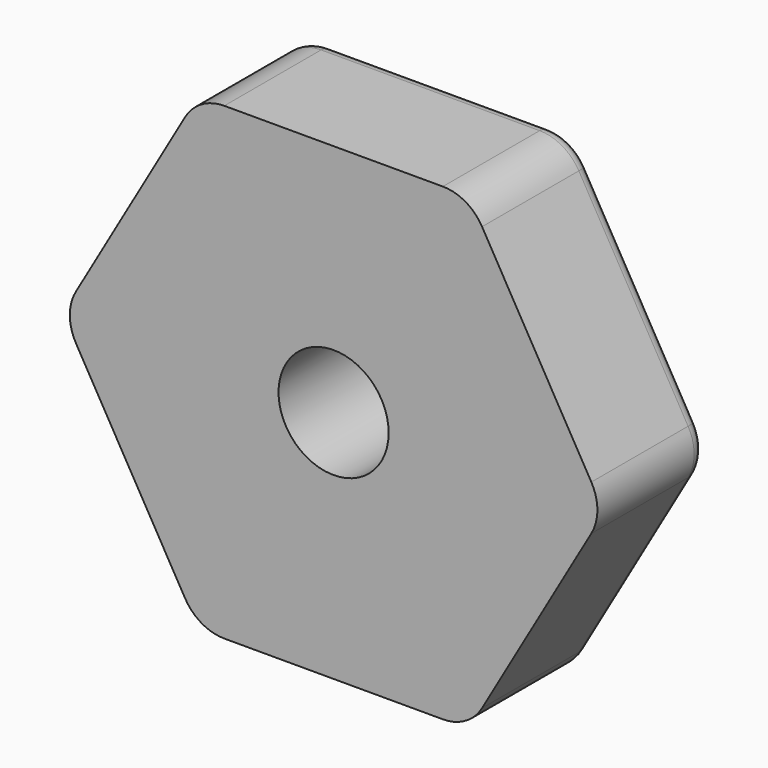
from build123d import *

# Parameters (mm, degrees)
F0_R          = 3.8735
F1_DEPTH      = 9.525
F2_R          = 6.4135
F3_DEPTH      = 6.35
F4_R          = 3.18262
F5_T1_DEPTH   = 5.9170310802
F5_T3_DEPTH   = 5.9170310802
F5_T5_DEPTH   = 5.9170310802
F5_T7_DEPTH   = 5.9170310802
F5_T9_DEPTH   = 5.9170310802
F5_T11_DEPTH  = 5.9170310802
F5_T13_DEPTH  = 5.9170310802
F5_T15_DEPTH  = 5.9170310802
F5_T17_DEPTH  = 5.9170310802
F5_T19_DEPTH  = 5.9170310802
F5_T21_DEPTH  = 5.9170310802
F5_T23_DEPTH  = 5.9170310802
F5_T26_ANGLE  = 76.4394190413
F5_T28_ANGLE  = 16.4394190413
F5_T30_ANGLE  = 16.4394190413
F5_T32_ANGLE  = 76.4394190413
F5_T34_ANGLE  = 76.4394190413
F5_T36_ANGLE  = 16.4394190413
F5_T38_ANGLE  = 16.4394190413
F5_T40_ANGLE  = 76.4394190413
F5_T42_ANGLE  = 76.4394190413
F5_T44_ANGLE  = 16.4394190413
F5_T46_ANGLE  = 16.4394190413
F5_T48_ANGLE  = 76.4394190413
F5_T51_DEPTH  = 15.3750269725
F5_T53_DEPTH  = 15.3750269725
F5_T55_DEPTH  = 15.3750269725
F5_T57_DEPTH  = 15.3750269725
F5_T59_DEPTH  = 15.3750269725
F5_T61_DEPTH  = 5.9170310802
F5_T63_DEPTH  = 5.9170310802
F5_T65_DEPTH  = 5.9170310802
F5_T67_DEPTH  = 5.9170310802
F5_T69_DEPTH  = 5.9170310802
F5_T71_DEPTH  = 5.9170310802
F5_T73_DEPTH  = 5.9170310802
F5_T75_DEPTH  = 5.9170310802
F5_T77_DEPTH  = 5.9170310802
F5_T79_DEPTH  = 5.9170310802
F5_T81_DEPTH  = 5.9170310802
F5_T83_DEPTH  = 5.9170310802
F5_T90_ANGLE  = 76.4394190413
F5_T92_ANGLE  = 60
F5_T94_ANGLE  = 60
F5_T96_ANGLE  = 60
F5_T98_ANGLE  = 60
F5_T100_ANGLE = 60
F5_T102_ANGLE = 60
F5_T104_ANGLE = 16.4394190413
F5_T106_ANGLE = 76.4394190413
F5_T108_ANGLE = 16.4394190413
F5_T110_ANGLE = 76.4394190413
F5_T112_ANGLE = 16.4394190413
F5_T114_ANGLE = 76.4394190413
F5_T116_ANGLE = 16.4394190413
F5_T118_ANGLE = 76.4394190413
F5_T120_ANGLE = 16.4394190413
F5_T122_ANGLE = 76.4394190413
F5_T124_ANGLE = 16.4394190413


# Not quite as in the source:
# - a fillet or chamfer that OpenCascade refuses, or shapes differently, is made with other operations: its cross-section is extruded or revolved along the edge and cut away or added


with BuildPart() as f1:
    # F0 (on Front) → F1 (new body)
    with BuildSketch(Plane.XZ):
        Polygon((19.05, 0), (9.525, 16.4977839421), (-9.525, 16.4977839421), (-19.05, 0), (-9.525, -16.4977839421), (9.525, -16.4977839421), align=None)
        Circle(F0_R, mode=Mode.SUBTRACT)
    extrude(amount=F1_DEPTH)

    # F2 (on face) → F3 (cut)
    with BuildSketch(Plane(origin=(0, 0, 0), x_dir=(-1, 0, 0), z_dir=(0, 1, 0))):
        Polygon((-12.0877954744, 6.978891971), (-17.5835303163, 0), (-12.0877954744, -6.978891971), (-8.7917651581, -15.2277839421), (0, -13.9577839421), (8.7917651581, -15.2277839421), (12.0877954744, -6.978891971), (17.5835303163, 0), (12.0877954744, 6.978891971), (8.7917651581, 15.2277839421), (0, 13.9577839421), (-8.7917651581, 15.2277839421), align=None)
        Circle(F2_R, mode=Mode.SUBTRACT)
    extrude(amount=-F3_DEPTH, mode=Mode.SUBTRACT)

    # F4
    f4_edges = [f1.edges().sort_by_distance(p)[0] for p in [
        (-17.58353, -3.175, 0),
        (-12.087795, -3.175, 6.978892),
        (-8.791765, -3.175, 15.227784),
        (0, -3.175, 13.957784),
        (8.791765, -3.175, 15.227784),
        (12.087795, -3.175, 6.978892),
        (17.58353, -3.175, 0),
        (12.087795, -3.175, -6.978892),
        (8.791765, -3.175, -15.227784),
        (0, -3.175, -13.957784),
        (-8.791765, -3.175, -15.227784),
        (-12.087795, -3.175, -6.978892),
        (-9.525, -4.7625, 16.497784),
        (9.525, -4.7625, 16.497784),
        (19.05, -4.7625, 0),
        (9.525, -4.7625, -16.497784),
        (-19.05, -4.7625, 0),
        (-9.525, -4.7625, -16.497784),
    ]]
    fillet(f4_edges, radius=F4_R)

    # F5: fillet of radius 1.016 on 29 edges, made by hand

    # F5_s2 → F5_t1 (join)
    with BuildSketch(Plane(origin=(-8.286299479, 0, 1.1969837853), x_dir=(0, 1, 0), z_dir=(0.9897271086, 0, -0.1429694044))):
        with BuildLine():
            ThreePointArc((-5.334, 13.8143971429), (-6.0524204897, 13.5168176326), (-6.35, 12.7983971429))
            Line((-6.35, 12.7983971429), (-6.35, 13.8143971429))
            Line((-6.35, 13.8143971429), (-5.334, 13.8143971429))
        make_face()
    extrude(amount=F5_T1_DEPTH)

    # F5_s4 → F5_t3 (join)
    with BuildSketch(Plane(origin=(0.9110263511, 0, 2.2800026795), x_dir=(0, 1, 0), z_dir=(0.3710484181, 0, 0.928613521))):
        with BuildLine():
            ThreePointArc((-5.334, 13.8143971429), (-6.0524204897, 13.5168176326), (-6.35, 12.7983971429))
            Line((-6.35, 12.7983971429), (-6.35, 13.8143971429))
            Line((-6.35, 13.8143971429), (-5.334, 13.8143971429))
        make_face()
    extrude(amount=F5_T3_DEPTH)

    # F5_s6 → F5_t5 (join)
    with BuildSketch(Plane(origin=(2.4300534167, 0, 0.3510293762), x_dir=(0, 1, 0), z_dir=(0.9897271086, 0, 0.1429694044))):
        with BuildLine():
            ThreePointArc((-5.334, 13.8143971429), (-6.0524204897, 13.5168176326), (-6.35, 12.7983971429))
            Line((-6.35, 12.7983971429), (-6.35, 13.8143971429))
            Line((-6.35, 13.8143971429), (-5.334, 13.8143971429))
        make_face()
    extrude(amount=F5_T5_DEPTH)

    # F5_s8 → F5_t7 (join)
    with BuildSketch(Plane(origin=(-5.1797681055, 0, -6.5776539596), x_dir=(0, 1, 0), z_dir=(0.6186786904, 0, 0.7856441167))):
        with BuildLine():
            ThreePointArc((-5.334, 13.8143971429), (-6.0524204897, 13.5168176326), (-6.35, 12.7983971429))
            Line((-6.35, 12.7983971429), (-6.35, 13.8143971429))
            Line((-6.35, 13.8143971429), (-5.334, 13.8143971429))
        make_face()
    extrude(amount=F5_T7_DEPTH)

    # F5_s10 → F5_t9 (join)
    with BuildSketch(Plane(origin=(-3.1065313735, 0, 7.7746377448), x_dir=(0, 1, 0), z_dir=(0.3710484181, 0, -0.928613521))):
        with BuildLine():
            ThreePointArc((-5.334, 13.8143971429), (-6.0524204897, 13.5168176326), (-6.35, 12.7983971429))
            Line((-6.35, 12.7983971429), (-6.35, 13.8143971429))
            Line((-6.35, 13.8143971429), (-5.334, 13.8143971429))
        make_face()
    extrude(amount=F5_T9_DEPTH)

    # F5_s12 → F5_t11 (join)
    with BuildSketch(Plane(origin=(-1.5190270656, 0, 1.9289733033), x_dir=(0, 1, 0), z_dir=(-0.6186786904, 0, 0.7856441167))):
        with BuildLine():
            ThreePointArc((-5.334, 13.8143971429), (-6.0524204897, 13.5168176326), (-6.35, 12.7983971429))
            Line((-6.35, 12.7983971429), (-6.35, 13.8143971429))
            Line((-6.35, 13.8143971429), (-5.334, 13.8143971429))
        make_face()
    extrude(amount=F5_T11_DEPTH)

    # F5_s14 → F5_t13 (join)
    with BuildSketch(Plane(origin=(1.5190270656, 0, -1.9289733033), x_dir=(0, 1, 0), z_dir=(0.6186786904, 0, -0.7856441167))):
        with BuildLine():
            ThreePointArc((-5.334, 13.8143971429), (-6.0524204897, 13.5168176326), (-6.35, 12.7983971429))
            Line((-6.35, 12.7983971429), (-6.35, 13.8143971429))
            Line((-6.35, 13.8143971429), (-5.334, 13.8143971429))
        make_face()
    extrude(amount=F5_T13_DEPTH)

    # F5_s16 → F5_t15 (join)
    with BuildSketch(Plane(origin=(3.1065313735, 0, -7.7746377448), x_dir=(0, 1, 0), z_dir=(-0.3710484181, 0, 0.928613521))):
        with BuildLine():
            ThreePointArc((-5.334, 13.8143971429), (-6.0524204897, 13.5168176326), (-6.35, 12.7983971429))
            Line((-6.35, 12.7983971429), (-6.35, 13.8143971429))
            Line((-6.35, 13.8143971429), (-5.334, 13.8143971429))
        make_face()
    extrude(amount=F5_T15_DEPTH)

    # F5_s18 → F5_t17 (join)
    with BuildSketch(Plane(origin=(5.1797681055, 0, 6.5776539596), x_dir=(0, 1, 0), z_dir=(-0.6186786904, 0, -0.7856441167))):
        with BuildLine():
            ThreePointArc((-5.334, 13.8143971429), (-6.0524204897, 13.5168176326), (-6.35, 12.7983971429))
            Line((-6.35, 12.7983971429), (-6.35, 13.8143971429))
            Line((-6.35, 13.8143971429), (-5.334, 13.8143971429))
        make_face()
    extrude(amount=F5_T17_DEPTH)

    # F5_s20 → F5_t19 (join)
    with BuildSketch(Plane(origin=(-2.4300534167, 0, -0.3510293762), x_dir=(0, 1, 0), z_dir=(-0.9897271086, 0, -0.1429694044))):
        with BuildLine():
            ThreePointArc((-5.334, 13.8143971429), (-6.0524204897, 13.5168176326), (-6.35, 12.7983971429))
            Line((-6.35, 12.7983971429), (-6.35, 13.8143971429))
            Line((-6.35, 13.8143971429), (-5.334, 13.8143971429))
        make_face()
    extrude(amount=F5_T19_DEPTH)

    # F5_s22 → F5_t21 (join)
    with BuildSketch(Plane(origin=(-0.9110263511, 0, -2.2800026795), x_dir=(0, 1, 0), z_dir=(-0.3710484181, 0, -0.928613521))):
        with BuildLine():
            ThreePointArc((-5.334, 13.8143971429), (-6.0524204897, 13.5168176326), (-6.35, 12.7983971429))
            Line((-6.35, 12.7983971429), (-6.35, 13.8143971429))
            Line((-6.35, 13.8143971429), (-5.334, 13.8143971429))
        make_face()
    extrude(amount=F5_T21_DEPTH)

    # F5_s24 → F5_t23 (join)
    with BuildSketch(Plane(origin=(8.286299479, 0, -1.1969837853), x_dir=(0, 1, 0), z_dir=(-0.9897271086, 0, 0.1429694044))):
        with BuildLine():
            ThreePointArc((-5.334, 13.8143971429), (-6.0524204897, 13.5168176326), (-6.35, 12.7983971429))
            Line((-6.35, 12.7983971429), (-6.35, 13.8143971429))
            Line((-6.35, 13.8143971429), (-5.334, 13.8143971429))
        make_face()
    extrude(amount=F5_T23_DEPTH)

    # F5_s25 → F5_t26 (revolve)
    with BuildSketch(Plane(origin=(3.1065313735, 0, 7.7746377448), x_dir=(0, 1, 0), z_dir=(-0.3710484181, 0, -0.928613521))):
        with BuildLine():
            ThreePointArc((-5.334, -13.8143971429), (-6.0524204897, -13.5168176326), (-6.35, -12.7983971429))
            Line((-6.35, -12.7983971429), (-6.35, -13.8143971429))
            Line((-6.35, -13.8143971429), (-5.334, -13.8143971429))
        make_face()
    revolve(axis=Axis((-6.7662806337, -6.35, 11.7195418358), (0, 1, 0)), revolution_arc=F5_T26_ANGLE)

    # F5_s27 → F5_t28 (revolve)
    with BuildSketch(Plane(origin=(2.4300534167, 0, 0.3510293762), x_dir=(0, 1, 0), z_dir=(0.9897271086, 0, 0.1429694044))):
        with BuildLine():
            ThreePointArc((-5.334, 13.8143971429), (-6.0524204897, 13.5168176326), (-6.35, 12.7983971429))
            Line((-6.35, 12.7983971429), (-6.35, 13.8143971429))
            Line((-6.35, 13.8143971429), (-5.334, 13.8143971429))
        make_face()
    revolve(axis=Axis((0, -6.35, 17.1734380072), (0, 1, 0)), revolution_arc=F5_T28_ANGLE)

    # F5_s29 → F5_t30 (revolve)
    with BuildSketch(Plane(origin=(0.9110263511, 0, 2.2800026795), x_dir=(0, 1, 0), z_dir=(0.3710484181, 0, 0.928613521))):
        with BuildLine():
            ThreePointArc((-5.334, 13.8143971429), (-6.0524204897, 13.5168176326), (-6.35, 12.7983971429))
            Line((-6.35, 12.7983971429), (-6.35, 13.8143971429))
            Line((-6.35, 13.8143971429), (-5.334, 13.8143971429))
        make_face()
    revolve(axis=Axis((-14.8726335846, -6.35, 8.5867190036), (0, 1, 0)), revolution_arc=F5_T30_ANGLE)

    # F5_s31 → F5_t32 (revolve)
    with BuildSketch(Plane(origin=(-3.1065313735, 0, 7.7746377448), x_dir=(0, 1, 0), z_dir=(0.3710484181, 0, -0.928613521))):
        with BuildLine():
            ThreePointArc((-5.334, 13.8143971429), (-6.0524204897, 13.5168176326), (-6.35, 12.7983971429))
            Line((-6.35, 12.7983971429), (-6.35, 13.8143971429))
            Line((-6.35, 13.8143971429), (-5.334, 13.8143971429))
        make_face()
    revolve(axis=Axis((6.7662806337, -6.35, 11.7195418358), (0, -1, 0)), revolution_arc=F5_T32_ANGLE)

    # F5_s33 → F5_t34 (revolve)
    with BuildSketch(Plane(origin=(-5.1797681055, 0, -6.5776539596), x_dir=(0, 1, 0), z_dir=(0.6186786904, 0, 0.7856441167))):
        with BuildLine():
            ThreePointArc((-5.334, 13.8143971429), (-6.0524204897, 13.5168176326), (-6.35, 12.7983971429))
            Line((-6.35, 12.7983971429), (-6.35, 13.8143971429))
            Line((-6.35, 13.8143971429), (-5.334, 13.8143971429))
        make_face()
    revolve(axis=Axis((-13.5325612674, -6.35, 0), (0, -1, 0)), revolution_arc=F5_T34_ANGLE)

    # F5_s35 → F5_t36 (revolve)
    with BuildSketch(Plane(origin=(1.5190270656, 0, -1.9289733033), x_dir=(0, 1, 0), z_dir=(0.6186786904, 0, -0.7856441167))):
        with BuildLine():
            ThreePointArc((-5.334, 13.8143971429), (-6.0524204897, 13.5168176326), (-6.35, 12.7983971429))
            Line((-6.35, 12.7983971429), (-6.35, 13.8143971429))
            Line((-6.35, 13.8143971429), (-5.334, 13.8143971429))
        make_face()
    revolve(axis=Axis((14.8726335846, -6.35, 8.5867190036), (0, 1, 0)), revolution_arc=F5_T36_ANGLE)

    # F5_s37 → F5_t38 (revolve)
    with BuildSketch(Plane(origin=(-1.5190270656, 0, 1.9289733033), x_dir=(0, 1, 0), z_dir=(-0.6186786904, 0, 0.7856441167))):
        with BuildLine():
            ThreePointArc((-5.334, 13.8143971429), (-6.0524204897, 13.5168176326), (-6.35, 12.7983971429))
            Line((-6.35, 12.7983971429), (-6.35, 13.8143971429))
            Line((-6.35, 13.8143971429), (-5.334, 13.8143971429))
        make_face()
    revolve(axis=Axis((-14.8726335846, -6.35, -8.5867190036), (0, 1, 0)), revolution_arc=F5_T38_ANGLE)

    # F5_s39 → F5_t40 (revolve)
    with BuildSketch(Plane(origin=(5.1797681055, 0, 6.5776539596), x_dir=(0, 1, 0), z_dir=(-0.6186786904, 0, -0.7856441167))):
        with BuildLine():
            ThreePointArc((-5.334, 13.8143971429), (-6.0524204897, 13.5168176326), (-6.35, 12.7983971429))
            Line((-6.35, 12.7983971429), (-6.35, 13.8143971429))
            Line((-6.35, 13.8143971429), (-5.334, 13.8143971429))
        make_face()
    revolve(axis=Axis((13.5325612674, -6.35, 0), (0, -1, 0)), revolution_arc=F5_T40_ANGLE)

    # F5_s41 → F5_t42 (revolve)
    with BuildSketch(Plane(origin=(3.1065313735, 0, -7.7746377448), x_dir=(0, 1, 0), z_dir=(-0.3710484181, 0, 0.928613521))):
        with BuildLine():
            ThreePointArc((-5.334, 13.8143971429), (-6.0524204897, 13.5168176326), (-6.35, 12.7983971429))
            Line((-6.35, 12.7983971429), (-6.35, 13.8143971429))
            Line((-6.35, 13.8143971429), (-5.334, 13.8143971429))
        make_face()
    revolve(axis=Axis((-6.7662806337, -6.35, -11.7195418358), (0, -1, 0)), revolution_arc=F5_T42_ANGLE)

    # F5_s43 → F5_t44 (revolve)
    with BuildSketch(Plane(origin=(-0.9110263511, 0, -2.2800026795), x_dir=(0, 1, 0), z_dir=(-0.3710484181, 0, -0.928613521))):
        with BuildLine():
            ThreePointArc((-5.334, 13.8143971429), (-6.0524204897, 13.5168176326), (-6.35, 12.7983971429))
            Line((-6.35, 12.7983971429), (-6.35, 13.8143971429))
            Line((-6.35, 13.8143971429), (-5.334, 13.8143971429))
        make_face()
    revolve(axis=Axis((14.8726335846, -6.35, -8.5867190036), (0, 1, 0)), revolution_arc=F5_T44_ANGLE)

    # F5_s45 → F5_t46 (revolve)
    with BuildSketch(Plane(origin=(-2.4300534167, 0, -0.3510293762), x_dir=(0, 1, 0), z_dir=(-0.9897271086, 0, -0.1429694044))):
        with BuildLine():
            ThreePointArc((-5.334, 13.8143971429), (-6.0524204897, 13.5168176326), (-6.35, 12.7983971429))
            Line((-6.35, 12.7983971429), (-6.35, 13.8143971429))
            Line((-6.35, 13.8143971429), (-5.334, 13.8143971429))
        make_face()
    revolve(axis=Axis((0, -6.35, -17.1734380072), (0, 1, 0)), revolution_arc=F5_T46_ANGLE)

    # F5_s47 → F5_t48 (revolve)
    with BuildSketch(Plane(origin=(8.286299479, 0, -1.1969837853), x_dir=(0, 1, 0), z_dir=(-0.9897271086, 0, 0.1429694044))):
        with BuildLine():
            ThreePointArc((-5.334, 13.8143971429), (-6.0524204897, 13.5168176326), (-6.35, 12.7983971429))
            Line((-6.35, 12.7983971429), (-6.35, 13.8143971429))
            Line((-6.35, 13.8143971429), (-5.334, 13.8143971429))
        make_face()
    revolve(axis=Axis((6.7662806337, -6.35, -11.7195418358), (0, -1, 0)), revolution_arc=F5_T48_ANGLE)

    # F5_s49 → F5_t50 (revolve)
    with BuildSketch(Plane.XY):
        with BuildLine():
            ThreePointArc((-7.4295, -6.35), (-6.7110795103, -6.0524204897), (-6.4135, -5.334))
            Line((-6.4135, -5.334), (-6.4135, -6.35))
            Line((-6.4135, -6.35), (-7.4295, -6.35))
        make_face()
    revolve(axis=Axis((0, -6.35, 0), (0, 1, 0)))

    # F5_s52 → F5_t51 (cut)
    with BuildSketch(Plane(origin=(-3.8437567431, 0, -6.657581971), x_dir=(0, 1, 0), z_dir=(0.5, 0, 0.8660254038))):
        with BuildLine():
            ThreePointArc((-1.016, -16.4977839421), (-0.2975795103, -16.2002044318), (0, -15.4817839421))
            Line((0, -15.4817839421), (0, -16.4977839421))
            Line((0, -16.4977839421), (-1.016, -16.4977839421))
        make_face()
    extrude(amount=F5_T51_DEPTH, mode=Mode.SUBTRACT)

    # F5_s54 → F5_t53 (cut)
    with BuildSketch(Plane(origin=(3.8437567431, 0, -6.657581971), x_dir=(0, 1, 0), z_dir=(-0.5, 0, 0.8660254038))):
        with BuildLine():
            ThreePointArc((0, -15.4817839421), (-0.2975795103, -16.2002044318), (-1.016, -16.4977839421))
            Line((-1.016, -16.4977839421), (0, -16.4977839421))
            Line((0, -16.4977839421), (0, -15.4817839421))
        make_face()
    extrude(amount=F5_T53_DEPTH, mode=Mode.SUBTRACT)

    # F5_s56 → F5_t55 (cut)
    with BuildSketch(Plane.YZ.offset(-7.6875134863)):
        with BuildLine():
            ThreePointArc((0, 15.4817839421), (-0.2975795103, 16.2002044318), (-1.016, 16.4977839421))
            Line((-1.016, 16.4977839421), (0, 16.4977839421))
            Line((0, 16.4977839421), (0, 15.4817839421))
        make_face()
        with BuildLine():
            ThreePointArc((0, -15.4817839421), (-0.2975795103, -16.2002044318), (-1.016, -16.4977839421))
            Line((-1.016, -16.4977839421), (0, -16.4977839421))
            Line((0, -16.4977839421), (0, -15.4817839421))
        make_face()
    extrude(amount=F5_T55_DEPTH, mode=Mode.SUBTRACT)

    # F5_s58 → F5_t57 (cut)
    with BuildSketch(Plane(origin=(3.8437567431, 0, 6.657581971), x_dir=(0, 1, 0), z_dir=(-0.5, 0, -0.8660254038))):
        with BuildLine():
            ThreePointArc((0, -15.4817839421), (-0.2975795103, -16.2002044318), (-1.016, -16.4977839421))
            Line((-1.016, -16.4977839421), (0, -16.4977839421))
            Line((0, -16.4977839421), (0, -15.4817839421))
        make_face()
    extrude(amount=F5_T57_DEPTH, mode=Mode.SUBTRACT)

    # F5_s60 → F5_t59 (cut)
    with BuildSketch(Plane(origin=(-3.8437567431, 0, 6.657581971), x_dir=(0, 1, 0), z_dir=(0.5, 0, -0.8660254038))):
        with BuildLine():
            ThreePointArc((0, -15.4817839421), (-0.2975795103, -16.2002044318), (-1.016, -16.4977839421))
            Line((-1.016, -16.4977839421), (0, -16.4977839421))
            Line((0, -16.4977839421), (0, -15.4817839421))
        make_face()
    extrude(amount=F5_T59_DEPTH, mode=Mode.SUBTRACT)

    # F5_s62 → F5_t61 (cut)
    with BuildSketch(Plane(origin=(5.1797681055, 0, 6.5776539596), x_dir=(0, 1, 0), z_dir=(-0.6186786904, 0, -0.7856441167))):
        with BuildLine():
            ThreePointArc((0, 14.8303971429), (-0.2975795103, 14.1119766532), (-1.016, 13.8143971429))
            Line((-1.016, 13.8143971429), (0, 13.8143971429))
            Line((0, 13.8143971429), (0, 14.8303971429))
        make_face()
    extrude(amount=F5_T61_DEPTH, mode=Mode.SUBTRACT)

    # F5_s64 → F5_t63 (cut)
    with BuildSketch(Plane(origin=(1.5190270656, 0, -1.9289733033), x_dir=(0, 1, 0), z_dir=(0.6186786904, 0, -0.7856441167))):
        with BuildLine():
            ThreePointArc((0, 14.8303971429), (-0.2975795103, 14.1119766532), (-1.016, 13.8143971429))
            Line((-1.016, 13.8143971429), (0, 13.8143971429))
            Line((0, 13.8143971429), (0, 14.8303971429))
        make_face()
    extrude(amount=F5_T63_DEPTH, mode=Mode.SUBTRACT)

    # F5_s66 → F5_t65 (cut)
    with BuildSketch(Plane(origin=(-3.1065313735, 0, 7.7746377448), x_dir=(0, 1, 0), z_dir=(0.3710484181, 0, -0.928613521))):
        with BuildLine():
            ThreePointArc((0, 14.8303971429), (-0.2975795103, 14.1119766532), (-1.016, 13.8143971429))
            Line((-1.016, 13.8143971429), (0, 13.8143971429))
            Line((0, 13.8143971429), (0, 14.8303971429))
        make_face()
    extrude(amount=F5_T65_DEPTH, mode=Mode.SUBTRACT)

    # F5_s68 → F5_t67 (cut)
    with BuildSketch(Plane(origin=(2.4300534167, 0, 0.3510293762), x_dir=(0, 1, 0), z_dir=(0.9897271086, 0, 0.1429694044))):
        with BuildLine():
            ThreePointArc((0, 14.8303971429), (-0.2975795103, 14.1119766532), (-1.016, 13.8143971429))
            Line((-1.016, 13.8143971429), (0, 13.8143971429))
            Line((0, 13.8143971429), (0, 14.8303971429))
        make_face()
    extrude(amount=F5_T67_DEPTH, mode=Mode.SUBTRACT)

    # F5_s70 → F5_t69 (cut)
    with BuildSketch(Plane(origin=(-8.286299479, 0, 1.1969837853), x_dir=(0, 1, 0), z_dir=(0.9897271086, 0, -0.1429694044))):
        with BuildLine():
            ThreePointArc((0, 14.8303971429), (-0.2975795103, 14.1119766532), (-1.016, 13.8143971429))
            Line((-1.016, 13.8143971429), (0, 13.8143971429))
            Line((0, 13.8143971429), (0, 14.8303971429))
        make_face()
    extrude(amount=F5_T69_DEPTH, mode=Mode.SUBTRACT)

    # F5_s72 → F5_t71 (cut)
    with BuildSketch(Plane(origin=(0.9110263511, 0, 2.2800026795), x_dir=(0, 1, 0), z_dir=(0.3710484181, 0, 0.928613521))):
        with BuildLine():
            ThreePointArc((0, 14.8303971429), (-0.2975795103, 14.1119766532), (-1.016, 13.8143971429))
            Line((-1.016, 13.8143971429), (0, 13.8143971429))
            Line((0, 13.8143971429), (0, 14.8303971429))
        make_face()
    extrude(amount=F5_T71_DEPTH, mode=Mode.SUBTRACT)

    # F5_s74 → F5_t73 (cut)
    with BuildSketch(Plane(origin=(-5.1797681055, 0, -6.5776539596), x_dir=(0, 1, 0), z_dir=(0.6186786904, 0, 0.7856441167))):
        with BuildLine():
            ThreePointArc((0, 14.8303971429), (-0.2975795103, 14.1119766532), (-1.016, 13.8143971429))
            Line((-1.016, 13.8143971429), (0, 13.8143971429))
            Line((0, 13.8143971429), (0, 14.8303971429))
        make_face()
    extrude(amount=F5_T73_DEPTH, mode=Mode.SUBTRACT)

    # F5_s76 → F5_t75 (cut)
    with BuildSketch(Plane(origin=(-1.5190270656, 0, 1.9289733033), x_dir=(0, 1, 0), z_dir=(-0.6186786904, 0, 0.7856441167))):
        with BuildLine():
            ThreePointArc((0, 14.8303971429), (-0.2975795103, 14.1119766532), (-1.016, 13.8143971429))
            Line((-1.016, 13.8143971429), (0, 13.8143971429))
            Line((0, 13.8143971429), (0, 14.8303971429))
        make_face()
    extrude(amount=F5_T75_DEPTH, mode=Mode.SUBTRACT)

    # F5_s78 → F5_t77 (cut)
    with BuildSketch(Plane(origin=(3.1065313735, 0, -7.7746377448), x_dir=(0, 1, 0), z_dir=(-0.3710484181, 0, 0.928613521))):
        with BuildLine():
            ThreePointArc((0, 14.8303971429), (-0.2975795103, 14.1119766532), (-1.016, 13.8143971429))
            Line((-1.016, 13.8143971429), (0, 13.8143971429))
            Line((0, 13.8143971429), (0, 14.8303971429))
        make_face()
    extrude(amount=F5_T77_DEPTH, mode=Mode.SUBTRACT)

    # F5_s80 → F5_t79 (cut)
    with BuildSketch(Plane(origin=(-2.4300534167, 0, -0.3510293762), x_dir=(0, 1, 0), z_dir=(-0.9897271086, 0, -0.1429694044))):
        with BuildLine():
            ThreePointArc((0, 14.8303971429), (-0.2975795103, 14.1119766532), (-1.016, 13.8143971429))
            Line((-1.016, 13.8143971429), (0, 13.8143971429))
            Line((0, 13.8143971429), (0, 14.8303971429))
        make_face()
    extrude(amount=F5_T79_DEPTH, mode=Mode.SUBTRACT)

    # F5_s82 → F5_t81 (cut)
    with BuildSketch(Plane(origin=(8.286299479, 0, -1.1969837853), x_dir=(0, 1, 0), z_dir=(-0.9897271086, 0, 0.1429694044))):
        with BuildLine():
            ThreePointArc((0, 14.8303971429), (-0.2975795103, 14.1119766532), (-1.016, 13.8143971429))
            Line((-1.016, 13.8143971429), (0, 13.8143971429))
            Line((0, 13.8143971429), (0, 14.8303971429))
        make_face()
    extrude(amount=F5_T81_DEPTH, mode=Mode.SUBTRACT)

    # F5_s84 → F5_t83 (cut)
    with BuildSketch(Plane(origin=(-0.9110263511, 0, -2.2800026795), x_dir=(0, 1, 0), z_dir=(-0.3710484181, 0, -0.928613521))):
        with BuildLine():
            ThreePointArc((0, 14.8303971429), (-0.2975795103, 14.1119766532), (-1.016, 13.8143971429))
            Line((-1.016, 13.8143971429), (0, 13.8143971429))
            Line((0, 13.8143971429), (0, 14.8303971429))
        make_face()
    extrude(amount=F5_T83_DEPTH, mode=Mode.SUBTRACT)

    # F5_s85 → F5_t86 (revolve, cut)
    with BuildSketch(Plane.XY):
        with BuildLine():
            ThreePointArc((-5.3975, 0), (-6.1159204897, -0.2975795103), (-6.4135, -1.016))
            Line((-6.4135, -1.016), (-6.4135, 0))
            Line((-6.4135, 0), (-5.3975, 0))
        make_face()
    revolve(axis=Axis((0, 0, 0), (0, 1, 0)), mode=Mode.SUBTRACT)

    # F5_s87 → F5_t88 (revolve, cut)
    with BuildSketch(Plane.XY):
        with BuildLine():
            ThreePointArc((3.8735, -1.016), (4.1710795103, -0.2975795103), (4.8895, 0))
            Line((4.8895, 0), (3.8735, 0))
            Line((3.8735, 0), (3.8735, -1.016))
        make_face()
    revolve(axis=Axis((0, 0, 0), (0, -1, 0)), mode=Mode.SUBTRACT)

    # F5_s89 → F5_t90 (revolve, cut)
    with BuildSketch(Plane(origin=(5.1797681055, 0, 6.5776539596), x_dir=(0, 1, 0), z_dir=(-0.6186786904, 0, -0.7856441167))):
        with BuildLine():
            ThreePointArc((0, 14.8303971429), (-0.2975795103, 14.1119766532), (-1.016, 13.8143971429))
            Line((-1.016, 13.8143971429), (0, 13.8143971429))
            Line((0, 13.8143971429), (0, 14.8303971429))
        make_face()
    revolve(axis=Axis((13.5325612674, 0, 0), (0, -1, 0)), revolution_arc=F5_T90_ANGLE, mode=Mode.SUBTRACT)

    # F5_s91 → F5_t92 (revolve, cut)
    with BuildSketch(Plane(origin=(3.8437567431, 0, 6.657581971), x_dir=(0, 1, 0), z_dir=(-0.5, 0, -0.8660254038))):
        with BuildLine():
            ThreePointArc((0, 15.4817839421), (-0.2975795103, 16.2002044318), (-1.016, 16.4977839421))
            Line((-1.016, 16.4977839421), (0, 16.4977839421))
            Line((0, 16.4977839421), (0, 15.4817839421))
        make_face()
    revolve(axis=Axis((15.3750269725, 0, 0), (0, -1, 0)), revolution_arc=F5_T92_ANGLE, mode=Mode.SUBTRACT)

    # F5_s93 → F5_t94 (revolve, cut)
    with BuildSketch(Plane(origin=(-3.8437567431, 0, 6.657581971), x_dir=(0, 1, 0), z_dir=(0.5, 0, -0.8660254038))):
        with BuildLine():
            ThreePointArc((0, 15.4817839421), (-0.2975795103, 16.2002044318), (-1.016, 16.4977839421))
            Line((-1.016, 16.4977839421), (0, 16.4977839421))
            Line((0, 16.4977839421), (0, 15.4817839421))
        make_face()
    revolve(axis=Axis((7.6875134863, 0, 13.3151639421), (0, -1, 0)), revolution_arc=F5_T94_ANGLE, mode=Mode.SUBTRACT)

    # F5_s95 → F5_t96 (revolve, cut)
    with BuildSketch(Plane.YZ.offset(-7.6875134863)):
        with BuildLine():
            ThreePointArc((0, 15.4817839421), (-0.2975795103, 16.2002044318), (-1.016, 16.4977839421))
            Line((-1.016, 16.4977839421), (0, 16.4977839421))
            Line((0, 16.4977839421), (0, 15.4817839421))
        make_face()
    revolve(axis=Axis((-7.6875134863, 0, 13.3151639421), (0, -1, 0)), revolution_arc=F5_T96_ANGLE, mode=Mode.SUBTRACT)

    # F5_s97 → F5_t98 (revolve, cut)
    with BuildSketch(Plane(origin=(-3.8437567431, 0, 6.657581971), x_dir=(0, 1, 0), z_dir=(0.5, 0, -0.8660254038))):
        with BuildLine():
            ThreePointArc((0, -15.4817839421), (-0.2975795103, -16.2002044318), (-1.016, -16.4977839421))
            Line((-1.016, -16.4977839421), (0, -16.4977839421))
            Line((0, -16.4977839421), (0, -15.4817839421))
        make_face()
    revolve(axis=Axis((-15.3750269725, 0, 0), (0, 1, 0)), revolution_arc=F5_T98_ANGLE, mode=Mode.SUBTRACT)

    # F5_s99 → F5_t100 (revolve, cut)
    with BuildSketch(Plane.YZ.offset(-7.6875134863)):
        with BuildLine():
            ThreePointArc((0, -15.4817839421), (-0.2975795103, -16.2002044318), (-1.016, -16.4977839421))
            Line((-1.016, -16.4977839421), (0, -16.4977839421))
            Line((0, -16.4977839421), (0, -15.4817839421))
        make_face()
    revolve(axis=Axis((-7.6875134863, 0, -13.3151639421), (0, 1, 0)), revolution_arc=F5_T100_ANGLE, mode=Mode.SUBTRACT)

    # F5_s101 → F5_t102 (revolve, cut)
    with BuildSketch(Plane(origin=(-3.8437567431, 0, -6.657581971), x_dir=(0, 1, 0), z_dir=(0.5, 0, 0.8660254038))):
        with BuildLine():
            ThreePointArc((0, -15.4817839421), (-0.2975795103, -16.2002044318), (-1.016, -16.4977839421))
            Line((-1.016, -16.4977839421), (0, -16.4977839421))
            Line((0, -16.4977839421), (0, -15.4817839421))
        make_face()
    revolve(axis=Axis((7.6875134863, 0, -13.3151639421), (0, 1, 0)), revolution_arc=F5_T102_ANGLE, mode=Mode.SUBTRACT)

    # F5_s103 → F5_t104 (revolve, cut)
    with BuildSketch(Plane(origin=(1.5190270656, 0, -1.9289733033), x_dir=(0, 1, 0), z_dir=(0.6186786904, 0, -0.7856441167))):
        with BuildLine():
            ThreePointArc((0, 14.8303971429), (-0.2975795103, 14.1119766532), (-1.016, 13.8143971429))
            Line((-1.016, 13.8143971429), (0, 13.8143971429))
            Line((0, 13.8143971429), (0, 14.8303971429))
        make_face()
    revolve(axis=Axis((14.8726335846, 0, 8.5867190036), (0, 1, 0)), revolution_arc=F5_T104_ANGLE, mode=Mode.SUBTRACT)

    # F5_s105 → F5_t106 (revolve, cut)
    with BuildSketch(Plane(origin=(-3.1065313735, 0, 7.7746377448), x_dir=(0, 1, 0), z_dir=(0.3710484181, 0, -0.928613521))):
        with BuildLine():
            ThreePointArc((0, 14.8303971429), (-0.2975795103, 14.1119766532), (-1.016, 13.8143971429))
            Line((-1.016, 13.8143971429), (0, 13.8143971429))
            Line((0, 13.8143971429), (0, 14.8303971429))
        make_face()
    revolve(axis=Axis((6.7662806337, 0, 11.7195418358), (0, -1, 0)), revolution_arc=F5_T106_ANGLE, mode=Mode.SUBTRACT)

    # F5_s107 → F5_t108 (revolve, cut)
    with BuildSketch(Plane(origin=(2.4300534167, 0, 0.3510293762), x_dir=(0, 1, 0), z_dir=(0.9897271086, 0, 0.1429694044))):
        with BuildLine():
            ThreePointArc((0, 14.8303971429), (-0.2975795103, 14.1119766532), (-1.016, 13.8143971429))
            Line((-1.016, 13.8143971429), (0, 13.8143971429))
            Line((0, 13.8143971429), (0, 14.8303971429))
        make_face()
    revolve(axis=Axis((0, 0, 17.1734380072), (0, 1, 0)), revolution_arc=F5_T108_ANGLE, mode=Mode.SUBTRACT)

    # F5_s109 → F5_t110 (revolve, cut)
    with BuildSketch(Plane(origin=(3.1065313735, 0, 7.7746377448), x_dir=(0, 1, 0), z_dir=(-0.3710484181, 0, -0.928613521))):
        with BuildLine():
            ThreePointArc((0, -14.8303971429), (-0.2975795103, -14.1119766532), (-1.016, -13.8143971429))
            Line((-1.016, -13.8143971429), (0, -13.8143971429))
            Line((0, -13.8143971429), (0, -14.8303971429))
        make_face()
    revolve(axis=Axis((-6.7662806337, 0, 11.7195418358), (0, 1, 0)), revolution_arc=F5_T110_ANGLE, mode=Mode.SUBTRACT)

    # F5_s111 → F5_t112 (revolve, cut)
    with BuildSketch(Plane(origin=(0.9110263511, 0, 2.2800026795), x_dir=(0, 1, 0), z_dir=(0.3710484181, 0, 0.928613521))):
        with BuildLine():
            ThreePointArc((0, 14.8303971429), (-0.2975795103, 14.1119766532), (-1.016, 13.8143971429))
            Line((-1.016, 13.8143971429), (0, 13.8143971429))
            Line((0, 13.8143971429), (0, 14.8303971429))
        make_face()
    revolve(axis=Axis((-14.8726335846, 0, 8.5867190036), (0, 1, 0)), revolution_arc=F5_T112_ANGLE, mode=Mode.SUBTRACT)

    # F5_s113 → F5_t114 (revolve, cut)
    with BuildSketch(Plane(origin=(-5.1797681055, 0, -6.5776539596), x_dir=(0, 1, 0), z_dir=(0.6186786904, 0, 0.7856441167))):
        with BuildLine():
            ThreePointArc((0, 14.8303971429), (-0.2975795103, 14.1119766532), (-1.016, 13.8143971429))
            Line((-1.016, 13.8143971429), (0, 13.8143971429))
            Line((0, 13.8143971429), (0, 14.8303971429))
        make_face()
    revolve(axis=Axis((-13.5325612674, 0, 0), (0, -1, 0)), revolution_arc=F5_T114_ANGLE, mode=Mode.SUBTRACT)

    # F5_s115 → F5_t116 (revolve, cut)
    with BuildSketch(Plane(origin=(-1.5190270656, 0, 1.9289733033), x_dir=(0, 1, 0), z_dir=(-0.6186786904, 0, 0.7856441167))):
        with BuildLine():
            ThreePointArc((0, 14.8303971429), (-0.2975795103, 14.1119766532), (-1.016, 13.8143971429))
            Line((-1.016, 13.8143971429), (0, 13.8143971429))
            Line((0, 13.8143971429), (0, 14.8303971429))
        make_face()
    revolve(axis=Axis((-14.8726335846, 0, -8.5867190036), (0, 1, 0)), revolution_arc=F5_T116_ANGLE, mode=Mode.SUBTRACT)

    # F5_s117 → F5_t118 (revolve, cut)
    with BuildSketch(Plane(origin=(3.1065313735, 0, -7.7746377448), x_dir=(0, 1, 0), z_dir=(-0.3710484181, 0, 0.928613521))):
        with BuildLine():
            ThreePointArc((0, 14.8303971429), (-0.2975795103, 14.1119766532), (-1.016, 13.8143971429))
            Line((-1.016, 13.8143971429), (0, 13.8143971429))
            Line((0, 13.8143971429), (0, 14.8303971429))
        make_face()
    revolve(axis=Axis((-6.7662806337, 0, -11.7195418358), (0, -1, 0)), revolution_arc=F5_T118_ANGLE, mode=Mode.SUBTRACT)

    # F5_s119 → F5_t120 (revolve, cut)
    with BuildSketch(Plane(origin=(-2.4300534167, 0, -0.3510293762), x_dir=(0, 1, 0), z_dir=(-0.9897271086, 0, -0.1429694044))):
        with BuildLine():
            ThreePointArc((0, 14.8303971429), (-0.2975795103, 14.1119766532), (-1.016, 13.8143971429))
            Line((-1.016, 13.8143971429), (0, 13.8143971429))
            Line((0, 13.8143971429), (0, 14.8303971429))
        make_face()
    revolve(axis=Axis((0, 0, -17.1734380072), (0, 1, 0)), revolution_arc=F5_T120_ANGLE, mode=Mode.SUBTRACT)

    # F5_s121 → F5_t122 (revolve, cut)
    with BuildSketch(Plane(origin=(8.286299479, 0, -1.1969837853), x_dir=(0, 1, 0), z_dir=(-0.9897271086, 0, 0.1429694044))):
        with BuildLine():
            ThreePointArc((0, 14.8303971429), (-0.2975795103, 14.1119766532), (-1.016, 13.8143971429))
            Line((-1.016, 13.8143971429), (0, 13.8143971429))
            Line((0, 13.8143971429), (0, 14.8303971429))
        make_face()
    revolve(axis=Axis((6.7662806337, 0, -11.7195418358), (0, -1, 0)), revolution_arc=F5_T122_ANGLE, mode=Mode.SUBTRACT)

    # F5_s123 → F5_t124 (revolve, cut)
    with BuildSketch(Plane(origin=(-0.9110263511, 0, -2.2800026795), x_dir=(0, 1, 0), z_dir=(-0.3710484181, 0, -0.928613521))):
        with BuildLine():
            ThreePointArc((0, 14.8303971429), (-0.2975795103, 14.1119766532), (-1.016, 13.8143971429))
            Line((-1.016, 13.8143971429), (0, 13.8143971429))
            Line((0, 13.8143971429), (0, 14.8303971429))
        make_face()
    revolve(axis=Axis((14.8726335846, 0, -8.5867190036), (0, 1, 0)), revolution_arc=F5_T124_ANGLE, mode=Mode.SUBTRACT)


solid = f1.part
